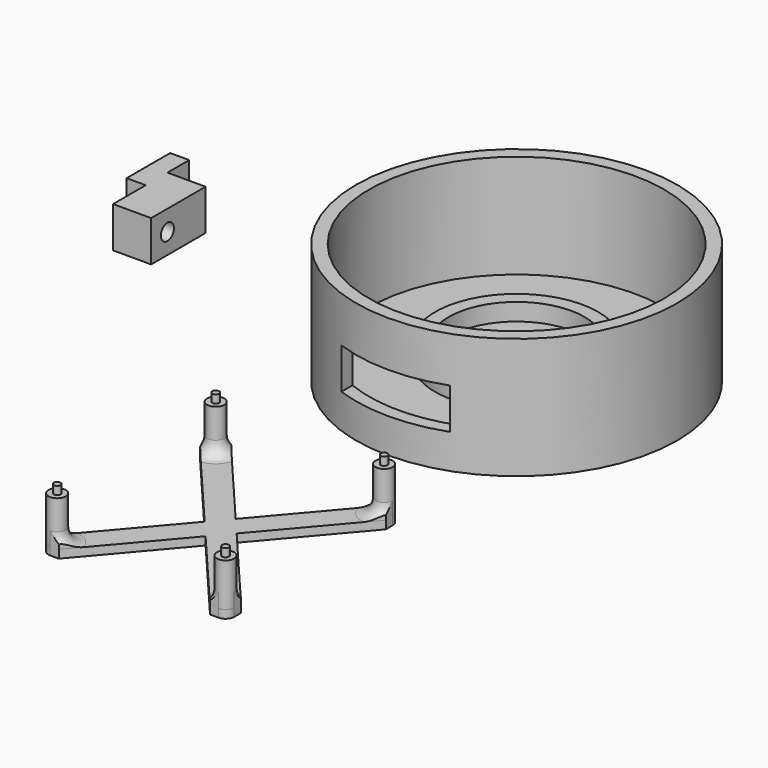
from build123d import *

# Parameters (mm, degrees)
F0_R          = 59
F1_DEPTH      = 6.35
F2_R          = 59
F2_R_2        = 54.25
F3_DEPTH      = 38.1
F4_R          = 30
F4_R_2        = 25
F5_DEPTH      = 6.35
F6_W          = 17.5801962614
F6_H          = 15
F7_DEPTH      = 20
F7_DEPTH_BACK = 20
F8_W          = 68.26
F8_H          = 79.2
F9_DEPTH      = 3
F11_DEPTH     = 25
F12_R         = 3.175
F13_DEPTH     = 15.875
F14_R         = 3.1749
F15_R         = 1.25
F16_DEPTH     = 3
F17_T4_ANGLE  = 270.0000007364
F17_T12_ANGLE = 90
F17_T18_ANGLE = 180
F17_T25_ANGLE = 270
F17_T33_ANGLE = 180
F17_T40_ANGLE = 90
F19_DEPTH     = 15
F20_R         = 3
F21_DEPTH     = 25


# Not quite as in the source:
# - a fillet or chamfer that OpenCascade refuses, or shapes differently, is made with other operations: its cross-section is extruded or revolved along the edge and cut away or added
# - a fillet or chamfer is up to 0.001 mm smaller than in the source, because OpenCascade refuses the exact size


with BuildPart() as f1:
    # F0 (on Top) → F1 (new body)
    with BuildSketch(Plane.XY):
        Circle(F0_R)
    extrude(amount=F1_DEPTH)

    # F2 (on face) → F3 (join)
    with BuildSketch(Plane.XY.offset(6.35)):
        Circle(F2_R)
        Circle(F2_R_2, mode=Mode.SUBTRACT)
    extrude(amount=F3_DEPTH)

    # F4 (on face) → F5 (join)
    with BuildSketch(Plane.XY.offset(6.35)):
        Circle(F4_R)
        Circle(F4_R_2, mode=Mode.SUBTRACT)
    extrude(amount=F5_DEPTH)

    # F6 (on Right) → F7 (cut, two sides)
    with BuildSketch(Plane.YZ) as f7_sk:
        with Locations((-53.9534389973, 20.2)):
            Rectangle(F6_W, F6_H)
    extrude(amount=F7_DEPTH, mode=Mode.SUBTRACT)
    extrude(f7_sk.sketch, amount=-F7_DEPTH_BACK, mode=Mode.SUBTRACT)


with BuildPart() as f9:
    # F8 (on Top) → F9 (new body)
    with BuildSketch(Plane.XY):
        with Locations((-5.9646429376, -128.5540193915)):
            Rectangle(F8_W, F8_H)
    extrude(amount=F9_DEPTH)

    # F10 (on face) → F11 (cut)
    with BuildSketch(Plane.XY.offset(3)):
        Polygon((-0.0914377214, -128.5540193915), (28.1653570624, -161.8040193915), (28.1653570624, -95.3040193915), align=None)
        Polygon((-33.7446429376, -88.9540193915), (-5.9646429376, -121.6429710956), (21.8153570624, -88.9540193915), align=None)
        Polygon((-33.7446429376, -168.1540193915), (21.8153570624, -168.1540193915), (-5.9646429376, -135.4650676875), align=None)
        Polygon((-40.0946429376, -161.8040193915), (-11.8378481538, -128.5540193915), (-40.0946429376, -95.3040193915), align=None)
    extrude(amount=-F11_DEPTH, mode=Mode.SUBTRACT)

    # F12 (on face) → F13 (join)
    with BuildSketch(Plane.XY.offset(3)):
        with Locations((-36.9196429376, -92.1290193915)):
            Circle(F12_R)
        with Locations((24.9903570624, -92.1290193915)):
            Circle(F12_R)
        with Locations((24.9903570624, -164.9790193915)):
            Circle(F12_R)
        with Locations((-36.9196429376, -164.9790193915)):
            Circle(F12_R)
    extrude(amount=F13_DEPTH)

    # F14 (radius 3.175 in the source; OpenCascade refuses exactly that, so slightly less here)
    f14_edges = [f9.edges().sort_by_distance(p)[0] for p in [
        (-40.094643, -168.154019, 1.5),
        (28.165357, -168.154019, 1.5),
        (28.165357, -88.954019, 1.5),
        (-40.094643, -88.954019, 1.5),
    ]]
    fillet(f14_edges, radius=F14_R)

    # F15 (on face) → F16 (join)
    with BuildSketch(Plane.XY.offset(18.875)):
        with Locations((24.9903570624, -164.9790193915)):
            Circle(F15_R)
        with Locations((24.9903570624, -92.1290193915)):
            Circle(F15_R)
        with Locations((-36.9196429376, -92.1290193915)):
            Circle(F15_R)
        with Locations((-36.9196429376, -164.9790193915)):
            Circle(F15_R)
    extrude(amount=F16_DEPTH)

    # F17: fillet of radius 5 on 6 edges, made by hand


with BuildPart() as f17_tool2:
    # F17_s3 → F17_t4 (revolve)
    with BuildSketch(Plane.XZ.offset(164.9790193915)):
        with BuildLine():
            ThreePointArc((33.1653570624, 3), (29.6298231565, 4.4644660941), (28.1653570624, 8))
            Line((28.1653570624, 8), (28.1653570624, 3))
            Line((28.1653570624, 3), (33.1653570624, 3))
        make_face()
    revolve(axis=Axis((24.9903570624, -164.9790193915, 3), (0, 0, 1)), revolution_arc=F17_T4_ANGLE)

    split(bisect_by=Plane(origin=(-70.308977279, -59.7505666897, 0), x_dir=(0, 0, 1), z_dir=(0.7620038344, 0.6475725105, 0)), keep=Keep.TOP)

    split(bisect_by=Plane.XZ.offset(168.1540193915), keep=Keep.BOTTOM)

    split(bisect_by=Plane.YZ.offset(28.1653570624), keep=Keep.BOTTOM)

    split(bisect_by=Plane(origin=(-63.4884258978, -53.954268323, 0), x_dir=(0, 0, 1), z_dir=(-0.7620038344, -0.6475725105, 0)), keep=Keep.TOP)


with BuildPart() as f9_1:
    add(f9.part)

    # F17_t1: union F17_tool2
    add(f17_tool2.part)


with BuildPart() as f17_tool10:
    # F17_s11 → F17_t12 (revolve)
    with BuildSketch(Plane.YZ.offset(-36.9196429376)):
        with BuildLine():
            ThreePointArc((-173.1540193915, 3), (-169.6184854856, 4.4644660941), (-168.1540193915, 8))
            Line((-168.1540193915, 8), (-168.1540193915, 3))
            Line((-168.1540193915, 3), (-173.1540193915, 3))
        make_face()
    revolve(axis=Axis((-36.9196429376, -164.9790193915, 3), (0, 0, 1)), revolution_arc=F17_T12_ANGLE)

    split(bisect_by=Plane.XZ.offset(168.1540193915), keep=Keep.BOTTOM)

    split(bisect_by=Plane(origin=(63.3822393005, -53.8640279354, 0), x_dir=(0, 0, 1), z_dir=(-0.7620038344, 0.6475725105, 0)), keep=Keep.TOP)


with BuildPart() as f9_2:
    add(f9_1.part)

    # F17_t9: union F17_tool10
    add(f17_tool10.part)


with BuildPart() as f17_tool16:
    # F17_s17 → F17_t18 (revolve)
    with BuildSketch(Plane.XZ.offset(164.9790193915)):
        with BuildLine():
            ThreePointArc((-28.7446429376, 3), (-32.2801768435, 4.4644660941), (-33.7446429376, 8))
            Line((-33.7446429376, 8), (-33.7446429376, 3))
            Line((-33.7446429376, 3), (-28.7446429376, 3))
        make_face()
    revolve(axis=Axis((-36.9196429376, -164.9790193915, 3), (0, 0, 1)), revolution_arc=F17_T18_ANGLE)

    split(bisect_by=Plane(origin=(63.3822393005, -53.8640279354, 0), x_dir=(0, 0, 1), z_dir=(-0.7620038344, 0.6475725105, 0)), keep=Keep.TOP)

    split(bisect_by=Plane.YZ.offset(-40.0946429376), keep=Keep.TOP)

    split(bisect_by=Plane(origin=(56.5616879193, -48.0677295688, 0), x_dir=(0, 0, 1), z_dir=(0.7620038344, -0.6475725105, 0)), keep=Keep.TOP)


with BuildPart() as f9_3:
    add(f9_2.part)

    # F17_t15: union F17_tool16
    add(f17_tool16.part)


with BuildPart() as f17_tool23:
    # F17_s24 → F17_t25 (revolve)
    with BuildSketch(Plane.YZ.offset(24.9903570624)):
        with BuildLine():
            ThreePointArc((-83.9540193915, 3), (-87.4895532975, 4.4644660941), (-88.9540193915, 8))
            Line((-88.9540193915, 8), (-88.9540193915, 3))
            Line((-88.9540193915, 3), (-83.9540193915, 3))
        make_face()
    revolve(axis=Axis((24.9903570624, -92.1290193915, 3), (0, 0, 1)), revolution_arc=F17_T25_ANGLE)

    split(bisect_by=Plane(origin=(56.5616879193, -48.0677295688, 0), x_dir=(0, 0, 1), z_dir=(0.7620038344, -0.6475725105, 0)), keep=Keep.TOP)

    split(bisect_by=Plane.XZ.offset(88.9540193915), keep=Keep.TOP)

    split(bisect_by=Plane(origin=(63.3822393005, -53.8640279354, 0), x_dir=(0, 0, 1), z_dir=(-0.7620038344, 0.6475725105, 0)), keep=Keep.TOP)

    split(bisect_by=Plane.YZ.offset(28.1653570624), keep=Keep.BOTTOM)


with BuildPart() as f9_4:
    add(f9_3.part)

    # F17_t22: union F17_tool23
    add(f17_tool23.part)


with BuildPart() as f17_tool31:
    # F17_s32 → F17_t33 (revolve)
    with BuildSketch(Plane.XZ.offset(92.1290193915)):
        with BuildLine():
            ThreePointArc((-45.0946429376, 3), (-41.5591090317, 4.4644660941), (-40.0946429376, 8))
            Line((-40.0946429376, 8), (-40.0946429376, 3))
            Line((-40.0946429376, 3), (-45.0946429376, 3))
        make_face()
    revolve(axis=Axis((-36.9196429376, -92.1290193915, 3), (0, 0, 1)), revolution_arc=F17_T33_ANGLE)

    split(bisect_by=Plane(origin=(-70.308977279, -59.7505666897, 0), x_dir=(0, 0, 1), z_dir=(0.7620038344, 0.6475725105, 0)), keep=Keep.TOP)

    split(bisect_by=Plane.YZ.offset(-40.0946429376), keep=Keep.TOP)

    split(bisect_by=Plane(origin=(-63.4884258978, -53.954268323, 0), x_dir=(0, 0, 1), z_dir=(-0.7620038344, -0.6475725105, 0)), keep=Keep.TOP)


with BuildPart() as f9_5:
    add(f9_4.part)

    # F17_t30: union F17_tool31
    add(f17_tool31.part)


with BuildPart() as f17_tool38:
    # F17_s39 → F17_t40 (revolve)
    with BuildSketch(Plane.XZ.offset(92.1290193915)):
        with BuildLine():
            ThreePointArc((-28.7446429376, 3), (-32.2801768435, 4.4644660941), (-33.7446429376, 8))
            Line((-33.7446429376, 8), (-33.7446429376, 3))
            Line((-33.7446429376, 3), (-28.7446429376, 3))
        make_face()
    revolve(axis=Axis((-36.9196429376, -92.1290193915, 3), (0, 0, 1)), revolution_arc=F17_T40_ANGLE)

    split(bisect_by=Plane.XZ.offset(88.9540193915), keep=Keep.TOP)

    split(bisect_by=Plane(origin=(-63.4884258978, -53.954268323, 0), x_dir=(0, 0, 1), z_dir=(-0.7620038344, -0.6475725105, 0)), keep=Keep.TOP)


with BuildPart() as f9_6:
    add(f9_5.part)

    # F17_t37: union F17_tool38
    add(f17_tool38.part)


with BuildPart() as f19:
    # F18 (on Top) → F19 (new body)
    with BuildSketch(Plane.XY):
        Polygon((-141.315436988, 26.2035948246), (-148.315436988, 26.2035948246), (-148.315436988, 6.2035948246), (-141.315436988, 6.2035948246), (-141.315436988, 16.2035948246), align=None)
        Polygon((-127.315436988, 16.2035948246), (-141.315436988, 16.2035948246), (-141.315436988, 6.2035948246), (-141.315436988, -8.7964051754), (-127.315436988, -8.7964051754), align=None)
    extrude(amount=F19_DEPTH)

    # F20 (on face) → F21 (cut)
    with BuildSketch(Plane(origin=(-141.315436988, 0, 0), x_dir=(0, -1, 0), z_dir=(-1, 0, 0))):
        with Locations((1.2964051754, 7.5)):
            Circle(F20_R)
    extrude(amount=-F21_DEPTH, mode=Mode.SUBTRACT)


solid = Compound([f1.part, f9_6.part, f19.part])
